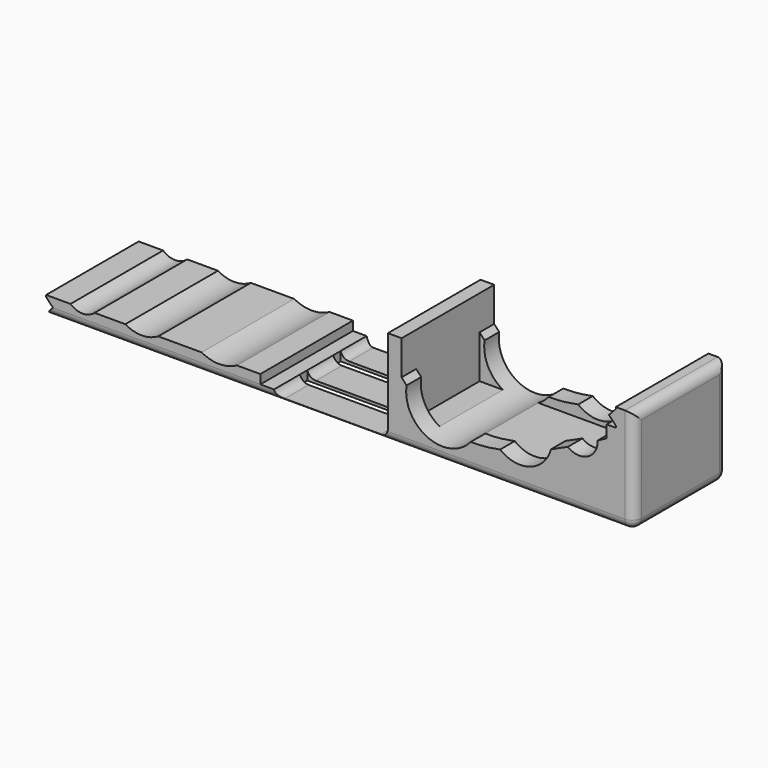
from build123d import *

# Parameters (mm, degrees)
F1_W          = 12.5
F1_H          = 0.3
F2_DEPTH      = 12.7
F5_START      = -1
F3_W          = 8.7
F3_H          = 6.7194561801
F5_DEPTH      = 22.5
F4_W          = 1.5
F4_H          = 1
F6_DEPTH      = 12.7
F4_H_2        = 10.5
F7_DEPTH      = 12.7
F8_W          = 12.5
F8_H          = 1
F9_DEPTH      = 0.3
F10_T1_DEPTH  = 3.5666666667
F10_T3_DEPTH  = 3.5666666667
F10_T5_DEPTH  = 3.5666666667
F10_T10_DEPTH = 8.5666666667
F10_T15_DEPTH = 8.5666666667
F10_T20_DEPTH = 8.5666666667
F10_T25_DEPTH = 8.5666666667
F10_T30_DEPTH = 8.3363626738
F10_T35_DEPTH = 8.3363626738
F10_T40_DEPTH = 8.3363626738
F10_T45_DEPTH = 8.3363626738
F11_T1_DEPTH  = 66
F11_T3_DEPTH  = 10.7
F11_T5_DEPTH  = 13
F11_T7_DEPTH  = 17.7
F11_S11_W     = 1
F11_S11_H     = 1
F11_T12_DEPTH = 1
F11_S17_W     = 1
F11_S17_H     = 1
F11_T18_DEPTH = 1


# Not quite as in the source:
# - a fillet or chamfer that OpenCascade refuses, or shapes differently, is made with other operations: its cross-section is extruded or revolved along the edge and cut away or added
# - a feature names something its author has since deleted; it is built from what else it names


with BuildPart() as f2:
    # F1 (on Front) → F2 (new body)
    with BuildSketch(Plane.XZ):
        with BuildLine():
            ThreePointArc((-25.9271243445, 2), (-27.25, 1.5), (-28.5728756555, 2))
            Line((-28.5728756555, 2), (-31.25, 2))
            Line((-31.25, 2), (-31.25, 0))
            Line((-31.25, 0), (-6.25, 0))
            Line((-6.25, 0), (-6.25, 0.3))
            Line((-6.25, 0.3), (-6.25, 2))
            Line((-6.25, 2), (-10.3135083269, 2))
            ThreePointArc((-10.3135083269, 2), (-12.25, 1.5), (-14.1864916731, 2))
            Line((-14.1864916731, 2), (-18.9472243623, 2))
            ThreePointArc((-18.9472243623, 2), (-20.75, 1.5), (-22.5527756377, 2))
            Line((-22.5527756377, 2), (-25.9271243445, 2))
        make_face()
        with Locations((0, 0.15)):
            Rectangle(F1_W, F1_H)
        with BuildLine():
            Line((6.25, 0.3), (6.25, 0))
            Line((6.25, 0), (31.25, 0))
            Line((31.25, 0), (31.25, 8.7194561801))
            add(Edge.make_bspline(
                [(29.2472199547, 7.6054156174), (29.8970928976, 7.9568787945), (30.5644371549, 8.3282256487), (31.25, 8.7194561801)],
                knots=[23.7294142738, 23.7294142738, 23.7294142738, 23.7294142738, 25, 25, 25, 25], degree=3))
            ThreePointArc((29.2472199547, 7.6054156174), (29.2493048679, 7.5527261345), (29.25, 7.5))
            ThreePointArc((29.25, 7.5), (28.112399222, 5.6954868851), (25.993732418, 5.9437892937))
            add(Edge.make_bspline(
                [(24.1320332758, 5.0989722973), (24.7343267633, 5.3573256266), (25.3545781422, 5.638931292), (25.993732418, 5.9437892937)],
                knots=[20.1331955968, 20.1331955968, 20.1331955968, 20.1331955968, 21.5072025076, 21.5072025076, 21.5072025076, 21.5072025076], degree=3))
            ThreePointArc((24.1320332758, 5.0989722973), (21.8431992343, 2.6751067033), (18.5625536561, 3.2677704173))
            add(Edge.make_bspline(
                [(15.3309754243, 2.9490020708), (16.3348264574, 2.926604162), (17.4079195378, 3.0328602775), (18.5625536561, 3.2677704173)],
                knots=[12.2186665261, 12.2186665261, 12.2186665261, 12.2186665261, 15.4506364332, 15.4506364332, 15.4506364332, 15.4506364332], degree=3))
            ThreePointArc((15.3309754243, 2.9490020708), (10.6056653115, 1.8536095338), (8.2983946259, 6.1203345608))
            add(Edge.make_bspline(
                [(6.25, 8.7194561801), (6.9059645215, 7.7244768722), (7.5846653889, 6.8581029991), (8.2983946259, 6.1203345608)],
                knots=[0, 0, 0, 0, 3.2313595313, 3.2313595313, 3.2313595313, 3.2313595313], degree=3))
            Line((6.25, 8.7194561801), (6.25, 0.3))
        make_face()
    extrude(amount=F2_DEPTH)

    # F3 (on face) → F5 (cut)
    with BuildSketch(Plane.YZ.offset(31.25).offset(F5_START)):
        with Locations((-6.35, 5.35972809)):
            Rectangle(F3_W, F3_H)
    extrude(amount=-F5_DEPTH, mode=Mode.SUBTRACT)

    # F4 (on Front) → F6 (cut, through all)
    with BuildSketch(Plane.XZ):
        with Locations((-7, 1.5)):
            Rectangle(F4_W, F4_H)
        Polygon((-30.5, 1), (-31.25, 1.8), (-31.25, 1), align=None)
        Polygon((-30.5, 1), (-31.25, 1), (-31.25, 0.2), align=None)
    extrude(amount=F6_DEPTH, mode=Mode.SUBTRACT)

    # F4 (on Front) → F7 (join, through all)
    with BuildSketch(Plane.XZ):
        Polygon((30.25, 0), (31.25, 0), (33.25, 0), (33.25, 11.5), (31.25, 11.5), (31.25, 11.3), (31.25, 10.5), (31.25, 9.7), (31.25, 9.5), (30.25, 9.5), align=None)
        with Locations((7, 5.25)):
            Rectangle(F4_W, F4_H_2)
        Polygon((30.5, 10.5), (31.25, 9.7), (31.25, 10.5), align=None)
        Polygon((31.25, 10.5), (31.25, 11.3), (30.5, 10.5), align=None)
    extrude(amount=F7_DEPTH)

    # F8 (on face) → F9 (cut, through all)
    with BuildSketch(Plane.XY.offset(0.3)):
        with Locations((0, -8.6333333333)):
            Rectangle(F8_W, F8_H)
        with Locations((0, -4.0666666667)):
            Rectangle(F8_W, F8_H)
    extrude(amount=-F9_DEPTH, mode=Mode.SUBTRACT)

    # F10: fillet of radius 1 on 6 edges, made by hand

    # F10_s2 → F10_t1 (join)
    with BuildSketch(Plane.XZ.offset(9.1333333333)):
        with BuildLine():
            ThreePointArc((6.25, 1.3), (5.9571067812, 0.5928932188), (5.25, 0.3))
            Line((5.25, 0.3), (6.25, 0.3))
            Line((6.25, 0.3), (6.25, 1.3))
        make_face()
        with BuildLine():
            ThreePointArc((-6.25, 1), (-5.8876687769, 0.4937742252), (-5.2960607986, 0.3))
            Line((-5.2960607986, 0.3), (-6.25, 0.3))
            Line((-6.25, 0.3), (-6.25, 1))
        make_face()
    extrude(amount=F10_T1_DEPTH)

    # F10_s4 → F10_t3 (join)
    with BuildSketch(Plane.XZ.offset(4.5666666667)):
        with BuildLine():
            ThreePointArc((6.25, 1.3), (5.9571067812, 0.5928932188), (5.25, 0.3))
            Line((5.25, 0.3), (6.25, 0.3))
            Line((6.25, 0.3), (6.25, 1.3))
        make_face()
        with BuildLine():
            ThreePointArc((-6.25, 1), (-5.8876687769, 0.4937742252), (-5.2960607986, 0.3))
            Line((-5.2960607986, 0.3), (-6.25, 0.3))
            Line((-6.25, 0.3), (-6.25, 1))
        make_face()
    extrude(amount=F10_T3_DEPTH)

    # F10_s6 → F10_t5 (join)
    with BuildSketch(Plane.XZ):
        with BuildLine():
            ThreePointArc((6.25, 1.3), (5.9571067812, 0.5928932188), (5.25, 0.3))
            Line((5.25, 0.3), (6.25, 0.3))
            Line((6.25, 0.3), (6.25, 1.3))
        make_face()
        with BuildLine():
            ThreePointArc((-5.2960607986, 0.3), (-5.8876687769, 0.4937742252), (-6.25, 1))
            Line((-6.25, 1), (-6.25, 0.3))
            Line((-6.25, 0.3), (-5.2960607986, 0.3))
        make_face()
    extrude(amount=F10_T5_DEPTH)


with BuildPart() as f10_tool8:
    # F10_s9 → F10_t10 (new body)
    with BuildSketch(Plane.XZ.offset(6.6333333333)):
        with BuildLine():
            ThreePointArc((6.25, 1.3), (5.9571067812, 0.5928932188), (5.25, 0.3))
            Line((5.25, 0.3), (6.25, 0.3))
            Line((6.25, 0.3), (6.25, 1.3))
        make_face()
    extrude(amount=F10_T10_DEPTH)

    split(bisect_by=Plane.XZ.offset(8.1333333333), keep=Keep.BOTTOM)


with BuildPart() as f2_1:
    add(f2.part)

    # F10_t7: union F10_tool8
    add(f10_tool8.part)


with BuildPart() as f10_tool13:
    # F10_s14 → F10_t15 (new body)
    with BuildSketch(Plane.XZ.offset(2.0666666667)):
        with BuildLine():
            ThreePointArc((6.25, 1.3), (5.9571067812, 0.5928932188), (5.25, 0.3))
            Line((5.25, 0.3), (6.25, 0.3))
            Line((6.25, 0.3), (6.25, 1.3))
        make_face()
    extrude(amount=F10_T15_DEPTH)

    split(bisect_by=Plane.XZ.offset(3.5666666667), keep=Keep.BOTTOM)


with BuildPart() as f2_2:
    add(f2_1.part)

    # F10_t12: union F10_tool13
    add(f10_tool13.part)


with BuildPart() as f10_tool18:
    # F10_s19 → F10_t20 (new body)
    with BuildSketch(Plane.XZ.offset(2.0666666667)):
        with BuildLine():
            ThreePointArc((6.25, 1.3), (5.9571067812, 0.5928932188), (5.25, 0.3))
            Line((5.25, 0.3), (6.25, 0.3))
            Line((6.25, 0.3), (6.25, 1.3))
        make_face()
    extrude(amount=F10_T20_DEPTH)

    split(bisect_by=Plane.XZ.offset(9.1333333333), keep=Keep.TOP)


with BuildPart() as f2_3:
    add(f2_2.part)

    # F10_t17: union F10_tool18
    add(f10_tool18.part)


with BuildPart() as f10_tool23:
    # F10_s24 → F10_t25 (new body)
    with BuildSketch(Plane.XZ.offset(-2.5)):
        with BuildLine():
            ThreePointArc((6.25, 1.3), (5.9571067812, 0.5928932188), (5.25, 0.3))
            Line((5.25, 0.3), (6.25, 0.3))
            Line((6.25, 0.3), (6.25, 1.3))
        make_face()
    extrude(amount=F10_T25_DEPTH)

    split(bisect_by=Plane.XZ.offset(4.5666666667), keep=Keep.TOP)


with BuildPart() as f2_4:
    add(f2_3.part)

    # F10_t22: union F10_tool23
    add(f10_tool23.part)


with BuildPart() as f10_tool28:
    # F10_s29 → F10_t30 (new body)
    with BuildSketch(Plane.XZ.offset(-2.3848480035)):
        with BuildLine():
            ThreePointArc((-5.2960607986, 0.3), (-5.8876687769, 0.4937742252), (-6.25, 1))
            Line((-6.25, 1), (-6.25, 0.3))
            Line((-6.25, 0.3), (-5.2960607986, 0.3))
        make_face()
    extrude(amount=F10_T30_DEPTH)

    split(bisect_by=Plane.XZ.offset(4.5666666667), keep=Keep.TOP)


with BuildPart() as f2_5:
    add(f2_4.part)

    # F10_t27: union F10_tool28
    add(f10_tool28.part)


with BuildPart() as f10_tool33:
    # F10_s34 → F10_t35 (new body)
    with BuildSketch(Plane.XZ.offset(2.1818186631)):
        with BuildLine():
            ThreePointArc((-6.25, 1), (-5.8876687769, 0.4937742252), (-5.2960607986, 0.3))
            Line((-5.2960607986, 0.3), (-6.25, 0.3))
            Line((-6.25, 0.3), (-6.25, 1))
        make_face()
    extrude(amount=F10_T35_DEPTH)

    split(bisect_by=Plane.XZ.offset(3.5666666667), keep=Keep.BOTTOM)


with BuildPart() as f2_6:
    add(f2_5.part)

    # F10_t32: union F10_tool33
    add(f10_tool33.part)


with BuildPart() as f10_tool38:
    # F10_s39 → F10_t40 (new body)
    with BuildSketch(Plane.XZ.offset(2.1818186631)):
        with BuildLine():
            ThreePointArc((-6.25, 1), (-5.8876687769, 0.4937742252), (-5.2960607986, 0.3))
            Line((-5.2960607986, 0.3), (-6.25, 0.3))
            Line((-6.25, 0.3), (-6.25, 1))
        make_face()
    extrude(amount=F10_T40_DEPTH)

    split(bisect_by=Plane.XZ.offset(9.1333333333), keep=Keep.TOP)


with BuildPart() as f2_7:
    add(f2_6.part)

    # F10_t37: union F10_tool38
    add(f10_tool38.part)


with BuildPart() as f10_tool43:
    # F10_s44 → F10_t45 (new body)
    with BuildSketch(Plane.XZ.offset(6.7484853298)):
        with BuildLine():
            ThreePointArc((-6.25, 1), (-5.8876687769, 0.4937742252), (-5.2960607986, 0.3))
            Line((-5.2960607986, 0.3), (-6.25, 0.3))
            Line((-6.25, 0.3), (-6.25, 1))
        make_face()
    extrude(amount=F10_T45_DEPTH)

    split(bisect_by=Plane.XZ.offset(8.1333333333), keep=Keep.BOTTOM)


with BuildPart() as f2_8:
    add(f2_7.part)

    # F10_t42: union F10_tool43
    add(f10_tool43.part)

    # F11: fillet of radius 1 on 6 edges, made by hand

    # F11_s2 → F11_t1 (cut)
    with BuildSketch(Plane.YZ.offset(-33.75)):
        with BuildLine():
            ThreePointArc((-1, 0), (-0.2928932188, 0.2928932188), (0, 1))
            Line((0, 1), (0, 0))
            Line((0, 0), (-1, 0))
        make_face()
        with BuildLine():
            ThreePointArc((-12.7, 1), (-12.4071067812, 0.2928932188), (-11.7, 0))
            Line((-11.7, 0), (-12.7, 0))
            Line((-12.7, 0), (-12.7, 1))
        make_face()
    extrude(amount=F11_T1_DEPTH, mode=Mode.SUBTRACT)

    # F11_s4 → F11_t3 (cut)
    with BuildSketch(Plane.XZ.offset(1)):
        with BuildLine():
            ThreePointArc((33.25, 1), (32.9571067812, 0.2928932188), (32.25, 0))
            Line((32.25, 0), (33.25, 0))
            Line((33.25, 0), (33.25, 1))
        make_face()
    extrude(amount=F11_T3_DEPTH, mode=Mode.SUBTRACT)

    # F11_s6 → F11_t5 (cut)
    with BuildSketch(Plane.XY.offset(1)):
        with BuildLine():
            ThreePointArc((32.25, -12.7), (32.9571067812, -12.4071067812), (33.25, -11.7))
            Line((33.25, -11.7), (33.25, -12.7))
            Line((33.25, -12.7), (32.25, -12.7))
        make_face()
        with BuildLine():
            ThreePointArc((33.25, -1), (32.9571067812, -0.2928932188), (32.25, 0))
            Line((32.25, 0), (33.25, 0))
            Line((33.25, 0), (33.25, -1))
        make_face()
    extrude(amount=F11_T5_DEPTH, mode=Mode.SUBTRACT)

    # F11_s8 → F11_t7 (cut)
    with BuildSketch(Plane.XZ.offset(-2.5)):
        with BuildLine():
            ThreePointArc((32.25, 11.5), (32.9571067812, 11.2071067812), (33.25, 10.5))
            Line((33.25, 10.5), (33.25, 11.5))
            Line((33.25, 11.5), (32.25, 11.5))
        make_face()
    extrude(amount=F11_T7_DEPTH, mode=Mode.SUBTRACT)


with BuildPart() as f11_tool10:
    # F11_s11 → F11_t12 (new body)
    with BuildSketch(Plane.XZ.offset(1)):
        with Locations((32.75, 0.5)):
            Rectangle(F11_S11_W, F11_S11_H)
    extrude(amount=-F11_T12_DEPTH)

    # F11_s13 → F11_t14 (revolve, cut)
    with BuildSketch(Plane(origin=(32.25, -1, 1), x_dir=(-0.7071067812, 0, 0.7071067812), z_dir=(-0.7071067812, 0, -0.7071067812))):
        with BuildLine():
            ThreePointArc((0, -1), (1, 0), (0, 1))
            Line((0, 1), (0, -1))
        make_face()
    revolve(axis=Axis((32.25, -1, 1), (0, 1, 0)), mode=Mode.SUBTRACT)


with BuildPart() as f2_9:
    add(f2_8.part)

    # F11_t9: cut F11_tool10
    add(f11_tool10.part, mode=Mode.SUBTRACT)


with BuildPart() as f11_tool16:
    # F11_s17 → F11_t18 (new body)
    with BuildSketch(Plane.XZ.offset(11.7)):
        with Locations((32.75, 0.5)):
            Rectangle(F11_S17_W, F11_S17_H)
    extrude(amount=F11_T18_DEPTH)

    # F11_s19 → F11_t20 (revolve, cut)
    with BuildSketch(Plane(origin=(32.25, -11.7, 1), x_dir=(-0.7071067812, 0, 0.7071067812), z_dir=(0.7071067812, 0, 0.7071067812))):
        with BuildLine():
            ThreePointArc((0, -1), (1, 0), (0, 1))
            Line((0, 1), (0, -1))
        make_face()
    revolve(axis=Axis((32.25, -11.7, 1), (0, -1, 0)), mode=Mode.SUBTRACT)


with BuildPart() as f2_10:
    add(f2_9.part)

    # F11_t15: cut F11_tool16
    add(f11_tool16.part, mode=Mode.SUBTRACT)


solid = f2_10.part
